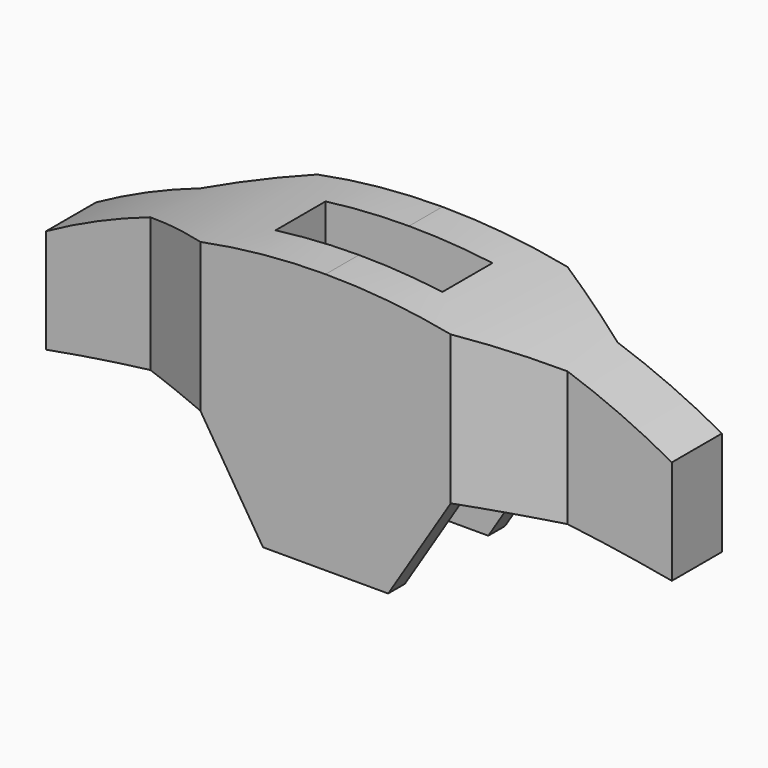
from build123d import *

# Parameters (mm, degrees)
F2_DEPTH    = 3
F3_DEPTH    = 5
F4_START    = 5
F4_DEPTH    = 2
F5_T4_DEPTH = 55.7006365314
F5_S5_R     = 165
F5_T6_DEPTH = 30
F5_S7_R     = 61.9381694392
F5_T8_DEPTH = 30
F6_DEPTH    = 3
F7_R        = 2.99999


# Not quite as in the source:
# - a fillet or chamfer that OpenCascade refuses, or shapes differently, is made with other operations: its cross-section is extruded or revolved along the edge and cut away or added
# - a fillet or chamfer is up to 0.001 mm smaller than in the source, because OpenCascade refuses the exact size
# - a feature names something its author has since deleted; it is built from what else it names


with BuildPart() as f2:
    # F1 (on Front) → F2 (new body)
    with BuildSketch(Plane.XZ):
        with BuildLine():
            ThreePointArc((-30, -2.7501926041), (-21.0318278303, -1.3459068092), (-12, -0.4369421772))
            Line((-12, -0.4369421772), (-12, 13.8264323737))
            ThreePointArc((-12, 13.8264323737), (-21.2558932775, 11.2384911254), (-30, 7.2498073959))
            Line((-30, 7.2498073959), (-30, -2.7501926041))
        make_face()
        with BuildLine():
            ThreePointArc((-12, -0.4369421772), (-6.0039761506, -0.1092717271), (0, 0))
            Line((0, 0), (0, 15))
            ThreePointArc((0, 15), (-6.028624656, 14.7059099053), (-12, 13.8264323737))
            Line((-12, 13.8264323737), (-12, -0.4369421772))
        make_face()
    extrude(amount=F2_DEPTH)

    # F1 (on Front) → F3 (join)
    with BuildSketch(Plane.XZ):
        with BuildLine():
            ThreePointArc((-12, -0.4369421772), (-6.0039761506, -0.1092717271), (0, 0))
            Line((0, 0), (0, 15))
            ThreePointArc((0, 15), (-6.028624656, 14.7059099053), (-12, 13.8264323737))
            Line((-12, 13.8264323737), (-12, -0.4369421772))
        make_face()
    extrude(amount=F3_DEPTH)

    # F1 (on Front) → F4 (join)
    with BuildSketch(Plane.XZ.offset(F4_START)):
        with BuildLine():
            Line((0, -10), (0, 0))
            ThreePointArc((0, 0), (-6.0039761506, -0.1092717271), (-12, -0.4369421772))
            Line((-12, -0.4369421772), (-6, -10))
            Line((-6, -10), (0, -10))
        make_face()
        with BuildLine():
            ThreePointArc((-12, -0.4369421772), (-6.0039761506, -0.1092717271), (0, 0))
            Line((0, 0), (0, 15))
            ThreePointArc((0, 15), (-6.028624656, 14.7059099053), (-12, 13.8264323737))
            Line((-12, 13.8264323737), (-12, -0.4369421772))
        make_face()
    extrude(amount=F4_DEPTH)

    # F5: chamfer of 4 x 8 on 1 edges, made by hand


with BuildPart() as f5_tool2:
    # F5_s3 → F5_t4 (new body)
    with BuildSketch(Plane.XY.offset(-21.1555731675)):
        with BuildLine():
            Line((-11.7137832989, -7.1431083506), (-20.2862167011, -2.8568916494))
            Line((-20.2862167011, -2.8568916494), (-20.2862167011, -2.6968916494))
            ThreePointArc((-20.2862167011, -2.6968916494), (-16.1431083506, -2.84), (-12, -2.84))
            Line((-12, -2.84), (-11.84, -3))
            ThreePointArc((-11.84, -3), (-11.84, -5.0715541753), (-11.5537832989, -7.1431083506))
            Line((-11.5537832989, -7.1431083506), (-11.7137832989, -7.1431083506))
        make_face()
    extrude(amount=F5_T4_DEPTH)

    # F5_s5 → F5_t6 (cut, symmetric)
    with BuildSketch(Plane.XZ.offset(4.9)):
        with Locations((0, -165)):
            Circle(F5_S5_R)
    extrude(amount=F5_T6_DEPTH, both=True, mode=Mode.SUBTRACT)

    # F5_s7 → F5_t8 (intersect, symmetric)
    with BuildSketch(Plane.XZ.offset(4.9)):
        with Locations((0, -46.9381694392)):
            Circle(F5_S7_R)
    extrude(amount=F5_T8_DEPTH, both=True, mode=Mode.INTERSECT)

    split(bisect_by=Plane.XZ.offset(7), keep=Keep.BOTTOM)


with BuildPart() as f2_1:
    add(f2.part)

    # F5_t1: union F5_tool2
    add(f5_tool2.part)

    # F0 (on Front) → F6 (cut)
    with BuildSketch(Plane.XZ):
        Polygon((0, -20), (0, 0), (0, 110), (-6, 110), (-6, 100), (-8, 100), (-8, 0), (-15, 0), (-15, -20), align=None)
    extrude(amount=F6_DEPTH, mode=Mode.SUBTRACT)

    # F7 (radius 3 in the source; OpenCascade refuses exactly that, so slightly less here)
    f7_edges = [f2_1.edges().sort_by_distance(p)[0] for p in [
        (-15, -3, -0.341616),
    ]]
    fillet(f7_edges, radius=F7_R)

    # F8: F2 across plane


with BuildPart() as f2_2:
    add(f2_1.part)
    add(f2_1.part.mirror(Plane.XZ))

    # F9: F2 across plane


with BuildPart() as f2_3:
    add(f2_2.part)
    add(f2_2.part.mirror(Plane.YZ))


solid = f2_3.part
